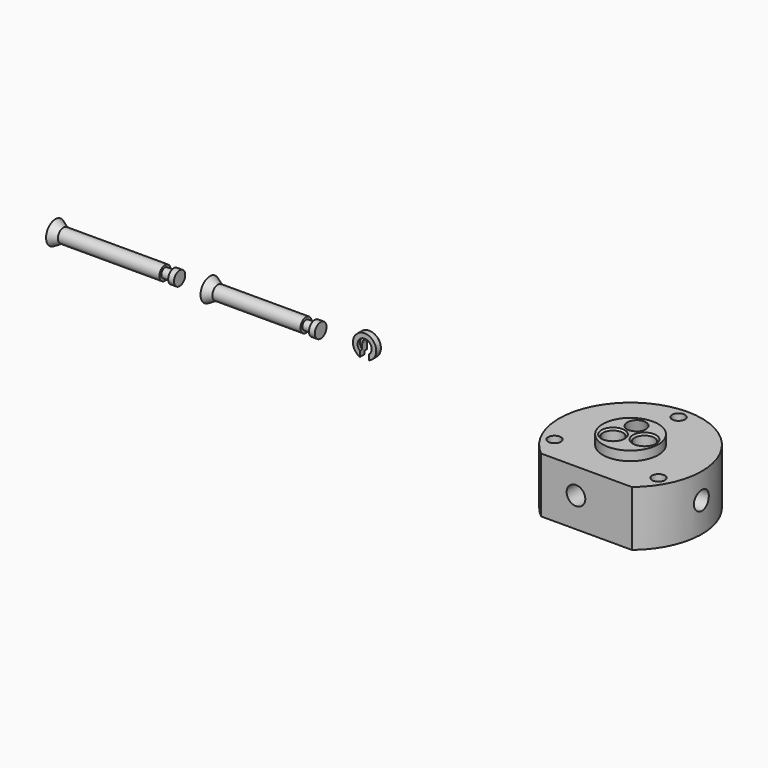
from build123d import *

# Parameters (mm, degrees)
F0_R            = 1.1
F0_R_2          = 4.75
F1_DEPTH        = 9.5
F2_DEPTH        = 1.6
F5_R            = 1.6
F6_DEPTH        = 14.5553932812
F8_R            = 2
F9_DEPTH        = 10
F10_R           = 3.25
F11_DEPTH       = 4
F13_D           = 3.4
F13_DEPTH       = 7.4
F13_CSINK_D     = 4
F13_CSINK_ANGLE = 90
F13_TIP         = 1.0214630523
F15_D           = 2.4
F17_D           = 3.2
F17_DEPTH       = 7.5
F17_TIP         = 0.9613769904
F19_D           = 2.4
F19_DEPTH       = 7.5
F19_TIP         = 0.7210327428
F22_D           = 3.2
F22_DEPTH       = 10
F22_TIP         = 0.9613769904
F26_DEPTH       = 1
F27_DEPTH       = 1.5
F28_DEPTH       = 0.5


# Not quite as in the source:
# - a feature of the source that left no trace in its solid (it failed there, or was rolled back) is left out


with BuildPart() as f1:
    # F0 (on Top) → F1 (new body)
    with BuildSketch(Plane.XY):
        with BuildLine():
            ThreePointArc((7.794870108, -9.45), (0, 12.25), (-7.794870108, -9.45))
            Line((-7.794870108, -9.45), (7.794870108, -9.45))
        make_face()
        with Locations((-8.920061659, -5.15)):
            Circle(F0_R, mode=Mode.SUBTRACT)
        Circle(F0_R_2, mode=Mode.SUBTRACT)
        with Locations((8.920061659, -5.15)):
            Circle(F0_R, mode=Mode.SUBTRACT)
        with Locations((0, 10.3)):
            Circle(F0_R, mode=Mode.SUBTRACT)
        Circle(F0_R_2)
    extrude(amount=-F1_DEPTH)

    # F0 (on Top) → F2 (join)
    with BuildSketch(Plane.XY):
        Circle(F0_R_2)
    extrude(amount=F2_DEPTH)

    # F5 (on face) → F6 (cut, through all)
    with BuildSketch(Plane(origin=(0.1177941054, -0.3141176144, 1.2520200421), x_dir=(0.9958620848, 0.0221147302, -0.0881455994), z_dir=(-0.0908774339, 0.2423398236, -0.9659258263))):
        with Locations((-0.9793015197, -2.7162409388)):
            Circle(F5_R)
    extrude(amount=F6_DEPTH, mode=Mode.SUBTRACT)

    # F8 (on face) → F9 (cut)
    with BuildSketch(Plane(origin=(-1.2453674026, 3.3209797402, -13.2368673522), x_dir=(0.9958620848, 0.0221147302, -0.0881455994), z_dir=(-0.0908774339, 0.2423398236, -0.9659258263))):
        with Locations((-0.984233483, -2.7172092824)):
            Circle(F8_R)
    extrude(amount=-F9_DEPTH, mode=Mode.SUBTRACT)

    # F10 (on face) → F11 (cut)
    with BuildSketch(Plane(origin=(-1.2453674026, 3.3209797402, -13.2368673522), x_dir=(0.9958620848, 0.0221147302, -0.0881455994), z_dir=(-0.0908774339, 0.2423398236, -0.9659258263))):
        with Locations((-0.9760213434, -2.7243471704)):
            Circle(F10_R)
    extrude(amount=-F11_DEPTH, mode=Mode.SUBTRACT)

    # F13
    with Locations(Plane.XY.offset(1.6)):
        with Locations((-1.8, -1.5), (2.4, 0)):
            CounterSinkHole(F13_D / 2, F13_CSINK_D / 2, depth=F13_DEPTH, counter_sink_angle=F13_CSINK_ANGLE)
            with Locations((0, 0, -(F13_DEPTH + F13_TIP / 2))):  # 118° drill point
                Cone(0, F13_D / 2, F13_TIP, mode=Mode.SUBTRACT)

    # F15 (through all)
    with Locations(Plane(origin=(0, 0, -9.5), x_dir=(1, 0, 0), z_dir=(0, 0, -1))):
        with Locations((2.4, 0), (-1.8, 1.5)):
            Hole(F15_D / 2)

    # F17
    with Locations(Plane.XZ.offset(9.45)):
        with Locations((-1.8, -4.4)):
            Hole(F17_D / 2, depth=F17_DEPTH)
            with Locations((0, 0, -(F17_DEPTH + F17_TIP / 2))):  # 118° drill point
                Cone(0, F17_D / 2, F17_TIP, mode=Mode.SUBTRACT)

    # F19
    with Locations(Plane(origin=(0, 0, -9.5), x_dir=(1, 0, 0), z_dir=(0, 0, -1))):
        with Locations((-7, 0)):
            Hole(F19_D / 2, depth=F19_DEPTH)
            with Locations((0, 0, -(F19_DEPTH + F19_TIP / 2))):  # 118° drill point
                Cone(0, F19_D / 2, F19_TIP, mode=Mode.SUBTRACT)

    # F22
    with Locations(Plane.YZ.offset(12.25)):
        with Locations((0, -4.4)):
            Hole(F22_D / 2, depth=F22_DEPTH)
            with Locations((0, 0, -(F22_DEPTH + F22_TIP / 2))):  # 118° drill point
                Cone(0, F22_D / 2, F22_TIP, mode=Mode.SUBTRACT)


with BuildPart() as f24:
    # F23 (on Front) → F24 (revolve)
    with BuildSketch(Plane.XZ):
        Polygon((-98.6498106364, 0), (-77.3498106364, 0), (-77.3498106364, 1.2), (-78.3498106364, 1.2), (-78.3498106364, 0.8), (-79.8498106364, 0.8), (-79.8498106364, 1.2), (-97.2641699903, 1.2), (-98.6498106364, 2), align=None)
    revolve(axis=Axis((-87.9998106364, 0, 0), (-1, 0, 0)))


with BuildPart() as f26:
    # F25 (on Front) → F26 (new body)
    with BuildSketch(Plane.XZ):
        with BuildLine():
            Line((-44.8178747118, -1.268857754), (-44.8178747118, -1.833030278))
            ThreePointArc((-44.8178747118, -1.833030278), (-45.6178747118, 2), (-46.4178747118, -1.833030278))
            Line((-46.4178747118, -1.833030278), (-46.4178747118, -1.268857754))
            ThreePointArc((-46.4178747118, -1.268857754), (-45.6178747118, 1.5), (-44.8178747118, -1.268857754))
        make_face()
        with BuildLine():
            Line((-44.8178747118, 0), (-44.8178747118, -0.894427191))
            ThreePointArc((-44.8178747118, -0.894427191), (-45.6178747118, 1.2), (-46.4178747118, -0.894427191))
            Line((-46.4178747118, -0.894427191), (-46.4178747118, 0))
            ThreePointArc((-46.4178747118, 0), (-45.6178747118, 0.8), (-44.8178747118, 0))
        make_face()
        with BuildLine():
            Line((-44.8178747118, -0.894427191), (-44.8178747118, -1.268857754))
            ThreePointArc((-44.8178747118, -1.268857754), (-45.6178747118, 1.5), (-46.4178747118, -1.268857754))
            Line((-46.4178747118, -1.268857754), (-46.4178747118, -0.894427191))
            ThreePointArc((-46.4178747118, -0.894427191), (-45.6178747118, 1.2), (-44.8178747118, -0.894427191))
        make_face()
    extrude(amount=-F26_DEPTH)

    # F25 (on Front) → F27 (join)
    with BuildSketch(Plane.XZ):
        with BuildLine():
            Line((-44.8178747118, 0), (-44.8178747118, -0.894427191))
            ThreePointArc((-44.8178747118, -0.894427191), (-45.6178747118, 1.2), (-46.4178747118, -0.894427191))
            Line((-46.4178747118, -0.894427191), (-46.4178747118, 0))
            ThreePointArc((-46.4178747118, 0), (-45.6178747118, 0.8), (-44.8178747118, 0))
        make_face()
        with BuildLine():
            Line((-44.8178747118, -0.894427191), (-44.8178747118, -1.268857754))
            ThreePointArc((-44.8178747118, -1.268857754), (-45.6178747118, 1.5), (-46.4178747118, -1.268857754))
            Line((-46.4178747118, -1.268857754), (-46.4178747118, -0.894427191))
            ThreePointArc((-46.4178747118, -0.894427191), (-45.6178747118, 1.2), (-44.8178747118, -0.894427191))
        make_face()
    extrude(amount=-F27_DEPTH)

    # F25 (on Front) → F28 (cut)
    with BuildSketch(Plane.XZ):
        with BuildLine():
            Line((-44.8178747118, 0), (-44.8178747118, -0.894427191))
            ThreePointArc((-44.8178747118, -0.894427191), (-45.6178747118, 1.2), (-46.4178747118, -0.894427191))
            Line((-46.4178747118, -0.894427191), (-46.4178747118, 0))
            ThreePointArc((-46.4178747118, 0), (-45.6178747118, 0.8), (-44.8178747118, 0))
        make_face()
    extrude(amount=-F28_DEPTH, mode=Mode.SUBTRACT)


with BuildPart() as f30:
    # F29 (on Front) → F30 (revolve)
    with BuildSketch(Plane.XZ):
        Polygon((-72.1521154046, 2), (-72.1521154046, 0), (-53.1521154046, 0), (-53.1521154046, 1.2581226385), (-54.1521154046, 1.2581226385), (-54.1521154046, 0.8), (-55.6521154046, 0.8), (-55.6521154046, 1.2), (-70.7664747586, 1.2), align=None)
    revolve(axis=Axis((-62.2638948262, 0, 0), (1, 0, 0)))


solid = Compound([f1.part, f24.part, f26.part, f30.part])
